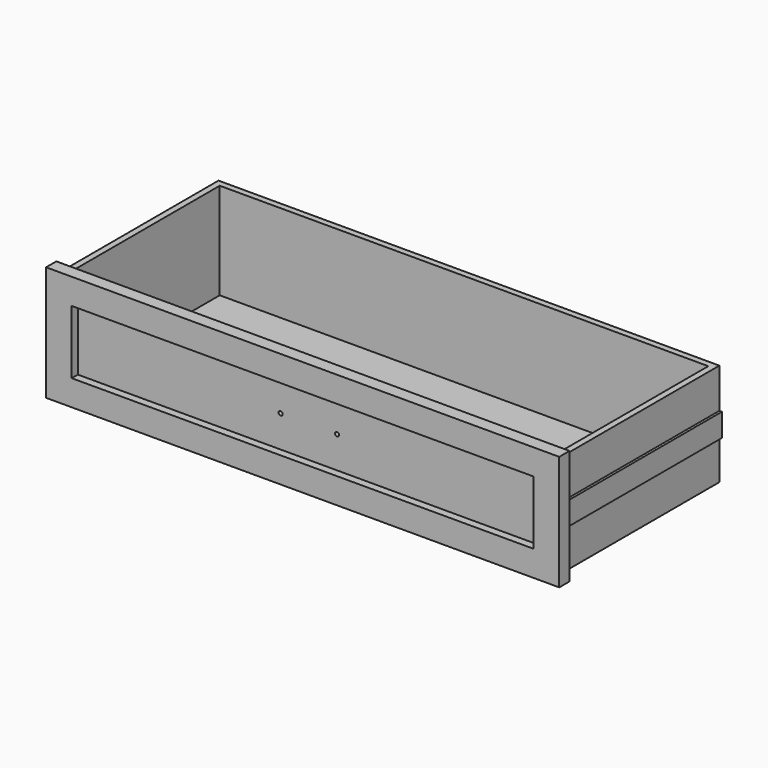
from build123d import *

# Parameters (mm, degrees)
F0_W      = 1000
F0_H      = 5.5340008238
F0_H_2    = 212.9319983523
F1_DEPTH  = 25
F2_W      = 900
F2_H      = 124
F3_DEPTH  = 15
F4_W      = 976
F4_H      = 200
F5_DEPTH  = 380
F6_T      = -12
F7_W      = 380
F7_H      = 45
F8_DEPTH  = 5
F9_W      = 380
F9_H      = 45
F10_DEPTH = 5
F11_R     = 4
F12_DEPTH = 12


# Not quite as in the source:
# - a shell that OpenCascade refuses in one call is made with other operations: the cavity is built on its own and cut out


with BuildPart() as f1:
    # F0 (on Front) → F1 (new body)
    with BuildSketch(Plane.XZ):
        with Locations((0, 109.2329995881)):
            Rectangle(F0_W, F0_H)
        Rectangle(F0_W, F0_H_2)
        with Locations((0, -109.2329995881)):
            Rectangle(F0_W, F0_H)
    extrude(amount=F1_DEPTH)

    # F2 (on face) → F3 (cut)
    with BuildSketch(Plane.XZ.offset(25)):
        Rectangle(F2_W, F2_H)
    extrude(amount=-F3_DEPTH, mode=Mode.SUBTRACT)

    # F4 (on face) → F5 (join)
    with BuildSketch(Plane(origin=(0, 0, 0), x_dir=(-1, 0, 0), z_dir=(0, 1, 0))):
        Rectangle(F4_W, F4_H)
    extrude(amount=F5_DEPTH)

    # F6: a shell. OpenCascade refuses it in one call, so the cavity is built on its own and cut out:
    # the body offset inwards by the wall thickness, plus a prism from it out through each open face.
    f6_core = offset(f1.part, amount=F6_T, kind=Kind.INTERSECTION, mode=Mode.PRIVATE)
    f6_exits = [f6_core.faces().sort_by_distance(p)[0] for p in [
        (0, 178, 88),
    ]]
    add(f6_core, mode=Mode.SUBTRACT)
    extrude(f6_exits, amount=-F6_T, mode=Mode.SUBTRACT)

    # F7 (on face) → F8 (join)
    with BuildSketch(Plane(origin=(-488, 0, 0), x_dir=(0, -1, 0), z_dir=(-1, 0, 0))):
        with Locations((-190, 0)):
            Rectangle(F7_W, F7_H)
    extrude(amount=F8_DEPTH)

    # F9 (on face) → F10 (join)
    with BuildSketch(Plane.YZ.offset(488)):
        with Locations((190, 0)):
            Rectangle(F9_W, F9_H)
    extrude(amount=F10_DEPTH)

    # F11 (on face) → F12 (cut, through all)
    with BuildSketch(Plane.XZ.offset(10)):
        with Locations((-55, 0)):
            Circle(F11_R)
        with BuildLine():
            ThreePointArc((59, 0), (55, 4), (51, 0))
            ThreePointArc((51, 0), (55, -4), (59, 0))
        make_face()
    extrude(amount=-F12_DEPTH, mode=Mode.SUBTRACT)


solid = f1.part
